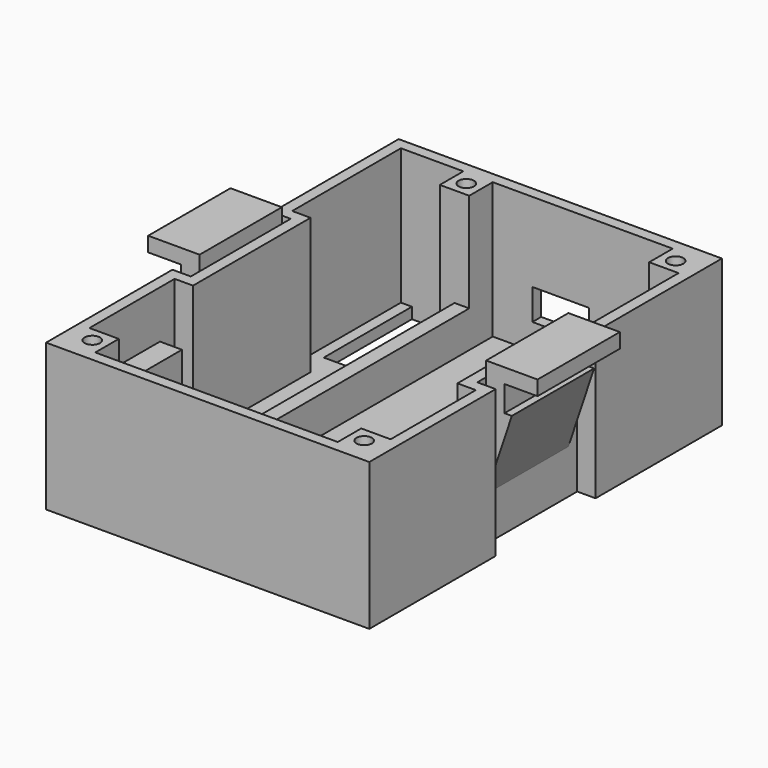
from build123d import *

# Parameters (mm, degrees)
F0_W      = 44
F0_H      = 60
F1_DEPTH  = 20
F2_W      = 2.5
F2_H      = 17
F3_DEPTH  = 20
F4_T      = -1.5
F5_W      = 5
F5_H      = 15
F6_DEPTH  = 2
F7_W      = 14
F7_H      = 2
F7_H_2    = 14
F8_DEPTH  = 7
F10_DEPTH = 14
F11_W     = 4
F11_H     = 4
F12_DEPTH = 18.5
F13_R     = 1.05
F14_DEPTH = 15
F15_W     = 7.7
F15_H     = 4.2
F16_DEPTH = 1.5
F17_W     = 2
F17_H     = 43.7
F17_H_2   = 39.7
F18_DEPTH = 5
F19_W     = 3
F19_H     = 10
F20_DEPTH = 12
F21_W     = 6
F21_H     = 2
F22_DEPTH = 10


# Not quite as in the source:
# - a pattern or mirror of a feature is missing from the dataset's text; its kind, count and spacing are read off the source's solid


with BuildPart() as f1:
    # F0 (on Top) → F1 (new body)
    with BuildSketch(Plane.XY):
        Rectangle(F0_W, F0_H)
    extrude(amount=F1_DEPTH)

    # F2 (on face) → F3 (cut)
    with BuildSketch(Plane.XY.offset(20)):
        with Locations((20.75, 0)):
            Rectangle(F2_W, F2_H)
        with Locations((-20.75, 0)):
            Rectangle(F2_W, F2_H)
    extrude(amount=-F3_DEPTH, mode=Mode.SUBTRACT)

    # F4
    f4_openings = [f1.faces().sort_by_distance(p)[0] for p in [
        (0, 0, 20),
    ]]
    offset(amount=F4_T, openings=f4_openings, kind=Kind.INTERSECTION)

    # F5 (on face) → F6 (cut)
    with BuildSketch(Plane(origin=(0, 0, 0), x_dir=(1, 0, 0), z_dir=(0, 0, -1))):
        with Locations((-16.5, -21)):
            Rectangle(F5_W, F5_H)
    extrude(amount=-F6_DEPTH, mode=Mode.SUBTRACT)

    # F7 (on face) → F8 (join)
    with BuildSketch(Plane.YZ.offset(19.5)):
        with Locations((0, 21)):
            Rectangle(F7_W, F7_H)
        with Locations((0, 13)):
            Rectangle(F7_W, F7_H_2)
    f8 = extrude(amount=F8_DEPTH)

    # F8_copies: F8 across plane
    add(f8.mirror(Plane(origin=(0, 0, 0), x_dir=(0, 0, -1), z_dir=(-1, 0, 0))))

    # F9 (on face) → F10 (cut)
    with BuildSketch(Plane.XZ.offset(7)):
        Polygon((23, 16.5), (19.5, 6), (26.5, 6), (26.5, 20), (22, 20), (22, 16.5), align=None)
    f10 = extrude(amount=-F10_DEPTH, mode=Mode.SUBTRACT)

    # F10_copies: F10 across plane
    add(f10.mirror(Plane(origin=(0, 0, 0), x_dir=(0, 0, -1), z_dir=(-1, 0, 0))), mode=Mode.SUBTRACT)

    # F11 (on face) → F12 (join, through all)
    with BuildSketch(Plane.XY.offset(1.5)):
        with Locations((18.5, 26.5)):
            Rectangle(F11_W, F11_H)
        with Locations((18.5, -26.5)):
            Rectangle(F11_W, F11_H)
        with Locations((-18.5, -26.5)):
            Rectangle(F11_W, F11_H)
        with Locations((-10, 26.5)):
            Rectangle(F11_W, F11_H)
    extrude(amount=F12_DEPTH)

    # F13 (on face) → F14 (cut)
    with BuildSketch(Plane.XY.offset(20)):
        with Locations((-10, 26.5)):
            Circle(F13_R)
        with Locations((18.5, 26.5)):
            Circle(F13_R)
        with Locations((18.5, -26.5)):
            Circle(F13_R)
        with Locations((-18.5, -26.5)):
            Circle(F13_R)
    extrude(amount=-F14_DEPTH, mode=Mode.SUBTRACT)

    # F15 (on face) → F16 (cut, through all)
    with BuildSketch(Plane.XZ.offset(-28.5)):
        with Locations((1.25, 7.1)):
            Rectangle(F15_W, F15_H)
    extrude(amount=-F16_DEPTH, mode=Mode.SUBTRACT)

    # F17 (on face) → F18 (join)
    with BuildSketch(Plane.XY.offset(1.5)):
        with Locations((11.6, 6.65)):
            Rectangle(F17_W, F17_H)
        Polygon((12.6, -15.2), (10.6, -15.2), (-8, -15.2), (-10, -15.2), (-10, -17.2), (12.6, -17.2), align=None)
        with Locations((-9, 4.65)):
            Rectangle(F17_W, F17_H_2)
    extrude(amount=F18_DEPTH)

    # F19 (on face) → F20 (join)
    with BuildSketch(Plane.XY.offset(1.5)):
        with Locations((19, 17.5)):
            Rectangle(F19_W, F19_H)
        with Locations((19, -17.5)):
            Rectangle(F19_W, F19_H)
        with Locations((-19, -17.5)):
            Rectangle(F19_W, F19_H)
    extrude(amount=F20_DEPTH)

    # F21 (on face) → F22 (cut)
    with BuildSketch(Plane.XY.offset(1.5)):
        with Locations((1.6, -16.2)):
            Rectangle(F21_W, F21_H)
    extrude(amount=F22_DEPTH, mode=Mode.SUBTRACT)


solid = f1.part
